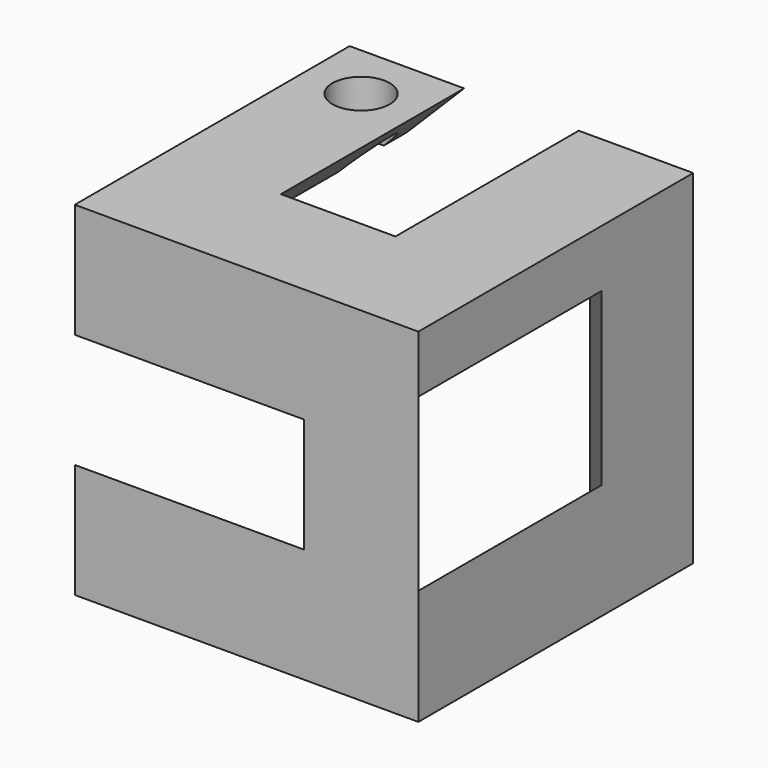
from build123d import *

# Parameters (mm, degrees)
F2_DEPTH = 2.5
F3_DEPTH = 2.5
F4_SIZE  = 2.49999
F8_DEPTH = 2.5
F9_SIZE  = 2.49999
F10_D    = 2.5


# Not quite as in the source:
# - a fillet or chamfer is up to 0.001 mm smaller than in the source, because OpenCascade refuses the exact size
# - a feature of the source that left no trace in its solid (it failed there, or was rolled back) is left out


with BuildPart() as f2:
    # F0 (on Front) → F2 (new body)
    with BuildSketch(Plane.XZ):
        Polygon((0, 7.5), (-15, 7.5), (-15, 2.5), (-5, 2.5), (-5, -2.5), (-15, -2.5), (-15, -7.5), (0, -7.5), align=None)
    extrude(amount=-F2_DEPTH)

    # F1 (on Right) → F3 (join)
    with BuildSketch(Plane.YZ):
        Polygon((15, -7.5), (15, -2.4617532641), (15, 5), (15, 7.5), (10, 7.5), (10, 5), (10, -2.4617532641), (0, -2.4617532641), (0, -7.5), align=None)
    extrude(amount=-F3_DEPTH)

    # F4 (call 1 of 3: OpenCascade refuses the feature's edges together) (size 2.5 in the source; OpenCascade refuses exactly that, so slightly less here)
    f4_edges = [f2.edges().sort_by_distance(p)[0] for p in [
        (0, 2.5, 2.519123),
    ]]
    chamfer(f4_edges, length=F4_SIZE)

    # F4#2 (call 2 of 3) (size 2.5 in the source; OpenCascade refuses exactly that, so slightly less here)
    f4_2_edges = [f2.edges().sort_by_distance(p)[0] for p in [
        (-10, 2.5, -2.5),
    ]]
    chamfer(f4_2_edges, length=F4_SIZE)

    # F4#3 (call 3 of 3) (size 2.5 in the source; OpenCascade refuses exactly that, so slightly less here)
    f4_3_edges = [f2.edges().sort_by_distance(p)[0] for p in [
        (-2.5, 10, 2.519123),
        (-2.5, 6.25, -2.461753),
    ]]
    chamfer(f4_3_edges, length=F4_SIZE)

    # F7 (on offset) → F8 (join)
    with BuildSketch(Plane.XY.offset(7.5)):
        Polygon((0, 0), (0, 15), (-5, 15), (-5, 5), (-10, 5), (-10, 15), (-15, 15), (-15, 0), align=None)
    extrude(amount=-F8_DEPTH)

    # F9 (size 2.5 in the source; OpenCascade refuses exactly that, so slightly less here)
    f9_edges = [f2.edges().sort_by_distance(p)[0] for p in [
        (-10, 10, 5),
    ]]
    chamfer(f9_edges, length=F9_SIZE)

    # F10 (through all)
    with Locations(Plane.XY.offset(7.5)):
        with Locations((-12.5, 12.5)):
            Hole(F10_D / 2)


solid = f2.part
